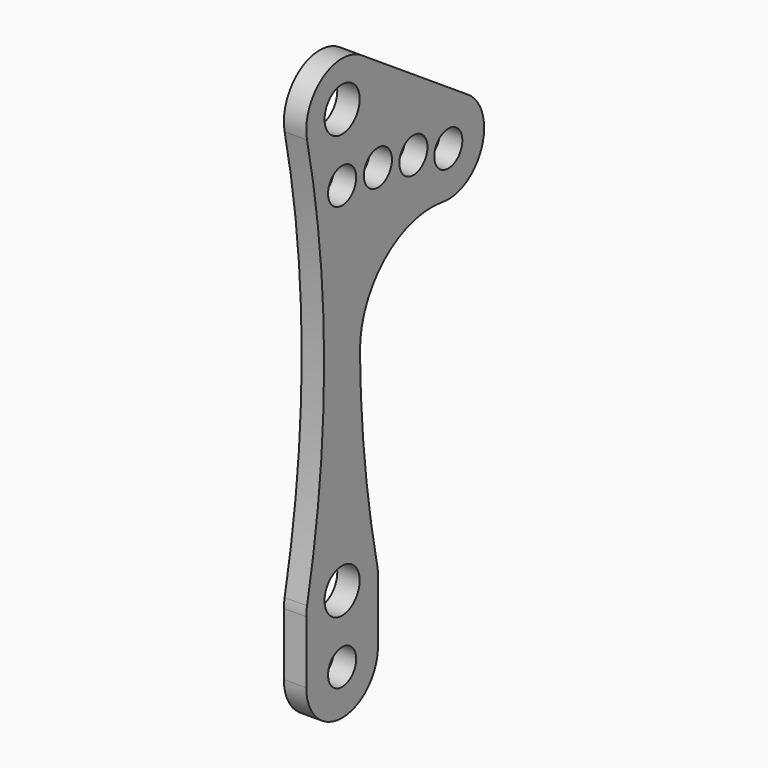
from build123d import *

# Parameters (mm, degrees)
F0_R     = 2.4892
F0_R_2   = 3.1115
F1_DEPTH = 3.175


# Not quite as in the source:
# - ends of sketch curves that miss each other by under 0.0002 mm in the source are joined


with BuildPart() as f1:
    # F0 (on Right) → F1 (new body)
    with BuildSketch(Plane.YZ):
        with BuildLine():
            Line((22.3326001159, -7.2636385381), (3.5237049527, 5.2826133121))
            ThreePointArc((3.5237049527, 5.2826133121), (-3.5587166415, 5.2590907831), (-6.2140895311, -1.3067483686))
            ThreePointArc((-6.2140895311, -1.3067483686), (-3.1920426976, -30.3630411987), (-6.2140895148, -59.419334071))
            ThreePointArc((-6.2140895148, -59.419334071), (-6.3159309852, -60.0691839024), (-6.35, -60.7260825175))
            Line((-6.35, -60.7260825175), (-6.35, -69.5833))
            ThreePointArc((-6.35, -69.5833), (0, -75.9333), (6.35, -69.5833))
            Line((6.35, -69.5833), (6.35, -60.7259096378))
            ThreePointArc((6.35, -60.7259096378), (6.3159401222, -60.069098879), (6.2141258668, -59.419334071))
            ThreePointArc((6.2141258668, -59.419334071), (4.0014684949, -45.5311698082), (3.1652638563, -31.4927325362))
            ThreePointArc((3.1652638563, -31.4927325362), (7.4831947902, -21.8210036968), (17.6308936292, -18.7860284798))
            ThreePointArc((17.6308936292, -18.7860284798), (24.6882615086, -14.9453248745), (22.3326001159, -7.2636385381))
        make_face()
        with Locations((0, -69.5833)):
            Circle(F0_R, mode=Mode.SUBTRACT)
        with Locations((0, -60.0583)):
            Circle(F0_R_2, mode=Mode.SUBTRACT)
        with Locations((0, -9.525)):
            Circle(F0_R, mode=Mode.SUBTRACT)
        Circle(F0_R_2, mode=Mode.SUBTRACT)
        with Locations((6.3411204926, -9.86069465)):
            Circle(F0_R, mode=Mode.SUBTRACT)
        with Locations((12.6288141023, -10.8677786001)):
            Circle(F0_R, mode=Mode.SUBTRACT)
        with Locations((18.8088951631, -12.5462518503)):
            Circle(F0_R, mode=Mode.SUBTRACT)
    extrude(amount=F1_DEPTH)


solid = f1.part
